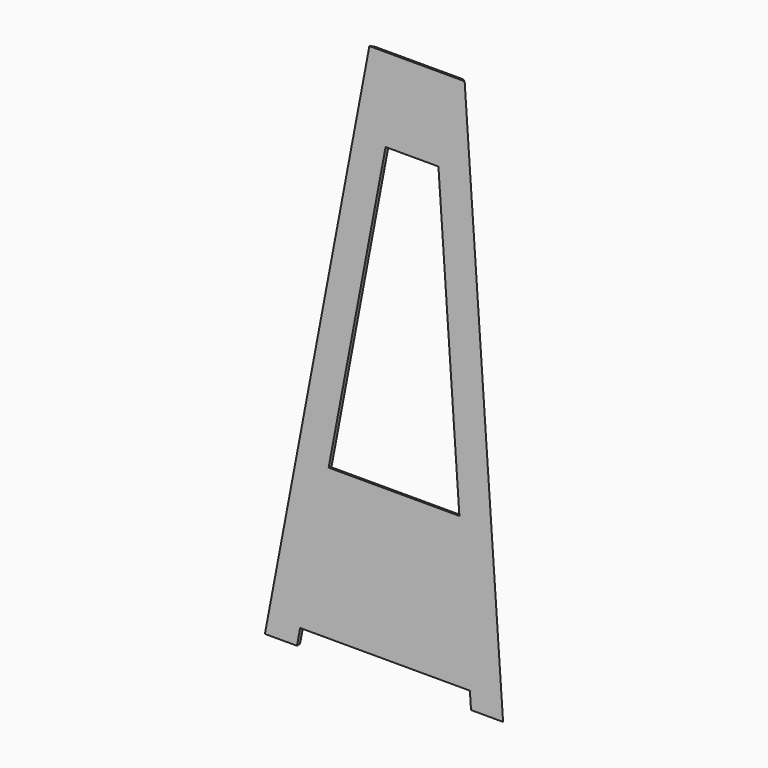
from build123d import *

# Parameters (mm, degrees)
F7_R      = 960.2431856589
F8_DEPTH  = 635.5163904251
F12_R     = 870.2287794889
F13_DEPTH = 25
F14_R     = 892.9375722879
F15_DEPTH = 25
F19_REACH = 935.9843056137
F20_DEPTH = 216.5073510461


with BuildPart() as f5:
    # F3 (on Top) → F5 section 0
    with BuildSketch(Plane.XY):
        Polygon((-375, -216.5063509461), (375, -216.5063509461), (0, 433.0127018922), align=None)
    # F4 (on line) → F5 section 1
    with BuildSketch(Plane.XY.offset(1650)):
        Polygon((-150, -86.6025403784), (150, -86.6025403784), (0, 173.2050807569), align=None)
    loft()

    # F7 (on face) → F8 (cut, through all)
    with BuildSketch(Plane(origin=(0, -203.2096543416, 15.9986111776), x_dir=(1, 0, 0), z_dir=(0, -0.9969151597, 0.078486714))):
        with Locations((0, 812.9688501358)):
            Circle(F7_R)
    extrude(amount=-F8_DEPTH, mode=Mode.SUBTRACT)

    # F12 (on face) → F13 (cut)
    with BuildSketch(Plane(origin=(0, 0, 0), x_dir=(0.8660254038, -0.5, 0), z_dir=(-0.5, -0.8660254038, 0))):
        with Locations((304.0688931942, 817.2121047974)):
            Circle(F12_R)
    extrude(amount=-F13_DEPTH, mode=Mode.SUBTRACT)

    # F14 (on face) → F15 (cut)
    with BuildSketch(Plane(origin=(0, 0, 0), x_dir=(-0.8660254038, -0.5, 0), z_dir=(-0.5, 0.8660254038, 0))):
        with Locations((291.6465699673, 811.1194968224)):
            Circle(F14_R)
    extrude(amount=F15_DEPTH, mode=Mode.SUBTRACT)

    f19_end = Plane(origin=(0, -155.5781982198, 697.4454188962), x_dir=(0, 0.078486714, 0.9969151597), z_dir=(0, 0.9969151597, -0.078486714))
    # F17 (on Front) → F19 (cut, up to a plane its end follows)
    with BuildSketch(Plane.XZ):
        Polygon((-181.3636363636, 1420), (181.3636363636, 1420), (179.7272727273, 1432), (-179.7272727273, 1432), align=None)
        Polygon((151.6363636364, 1638), (150, 1650), (-150, 1650), (-151.6363636364, 1638), align=None)
        Polygon((308.4545454545, 488), (306.8181818182, 500), (-306.8181818182, 500), (-308.4545454545, 488), align=None)
        Polygon((-365.4545454545, 70), (365.4545454545, 70), (363.8181818182, 82), (-363.8181818182, 82), align=None)
    f19_long = extrude(amount=F19_REACH, mode=Mode.PRIVATE)
    add(split(f19_long, bisect_by=f19_end, keep=Keep.TOP, mode=Mode.PRIVATE), mode=Mode.SUBTRACT)

    # F16 (on Front) → F20 (cut, through all)
    with BuildSketch(Plane.XZ):
        Polygon((-267.2563485856, 50), (-274.0745304038, 0), (274.0745304038, 0), (267.2563485856, 50), align=None)
        Polygon((-205.8927122219, 500), (205.8927122219, 500), (83.1654394947, 1400), (-83.1654394947, 1400), align=None)
    extrude(amount=F20_DEPTH, mode=Mode.SUBTRACT)


solid = f5.part
